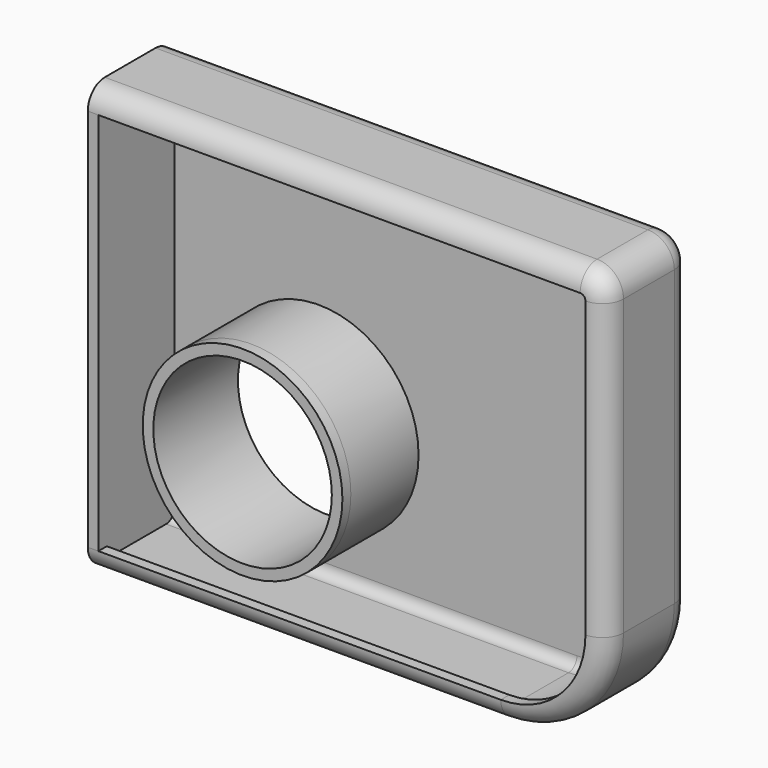
from build123d import *

# Parameters (mm, degrees)
F0_R     = 21.4314801072
F1_DEPTH = 12.7
F2_R     = 5.08
F3_T     = -2.54


# Not quite as in the source:
# - a shell that OpenCascade refuses in one call is made with other operations: the cavity is built on its own and cut out


with BuildPart() as f1:
    # F0 (on Front) → F1 (new body, symmetric)
    with BuildSketch(Plane.XZ):
        with BuildLine():
            Line((0, 102.3351529121), (0, 0))
            Line((0, 0), (99.1575824261, 0))
            ThreePointArc((99.1575824261, 0), (117.1180946682, 7.4394877579), (124.5575824261, 25.4))
            Line((124.5575824261, 25.4), (124.5575824261, 95.9851529121))
            ThreePointArc((124.5575824261, 95.9851529121), (122.6977104866, 100.4752809727), (118.2075824261, 102.3351529121))
            Line((118.2075824261, 102.3351529121), (0, 102.3351529121))
        make_face()
        with Locations((37.157318583, 35.142709024)):
            Circle(F0_R, mode=Mode.SUBTRACT)
    extrude(amount=F1_DEPTH, both=True)

    # F2
    f2_edges = [f1.edges().sort_by_distance(p)[0] for p in [
        (59.103791, 12.7, 102.335153),
        (59.103791, -12.7, 102.335153),
    ]]
    fillet(f2_edges, radius=F2_R)

    # F3: a shell. OpenCascade refuses it in one call, so the cavity is built on its own and cut out:
    # the body offset inwards by the wall thickness, plus a prism from it out through each open face.
    f3_core = offset(f1.part, amount=F3_T, mode=Mode.PRIVATE)
    f3_exits = [f3_core.faces().sort_by_distance(p)[0] for p in [
        (65.31507, -10.16, 54.836293),
    ]]
    add(f3_core, mode=Mode.SUBTRACT)
    extrude(f3_exits, amount=-F3_T, mode=Mode.SUBTRACT)


solid = f1.part
